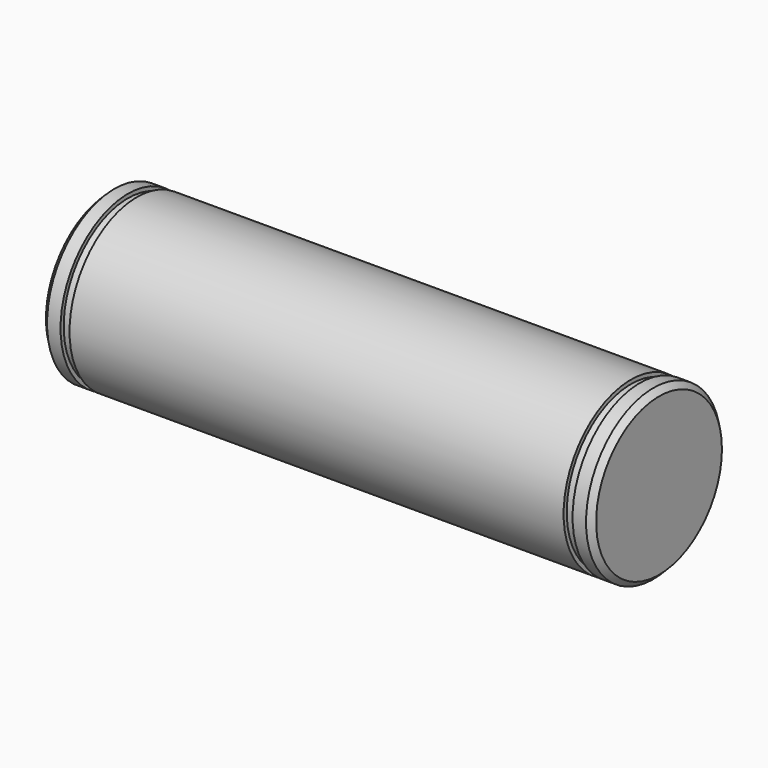
from build123d import *

# Parameters (mm, degrees)
F0_R     = 15
F1_DEPTH = 49
F3_R     = 17.9592935662
F3_R_2   = 14.3
F4_DEPTH = 1.6
F5_SIZE  = 1


# Not quite as in the source:
# - a pattern or mirror of a feature is missing from the dataset's text; its kind, count and spacing are read off the source's solid


with BuildPart() as f1:
    # F0 (on Right) → F1 (new body, symmetric)
    with BuildSketch(Plane.YZ):
        Circle(F0_R)
    extrude(amount=F1_DEPTH, both=True)

    # F3 (on offset) → F4 (cut)
    with BuildSketch(Plane.YZ.offset(44)):
        Circle(F3_R)
        Circle(F3_R_2, mode=Mode.SUBTRACT)
    f4 = extrude(amount=F4_DEPTH, mode=Mode.SUBTRACT)

    # F4_copies: F4 across plane
    add(f4.mirror(Plane(origin=(0, 0, 0), x_dir=(0, 0, -1), z_dir=(-1, 0, 0))), mode=Mode.SUBTRACT)

    # F5
    f5_edges = [f1.edges().sort_by_distance(p)[0] for p in [
        (-49, -15, 0),
        (49, -15, 0),
    ]]
    chamfer(f5_edges, length=F5_SIZE)


solid = f1.part
